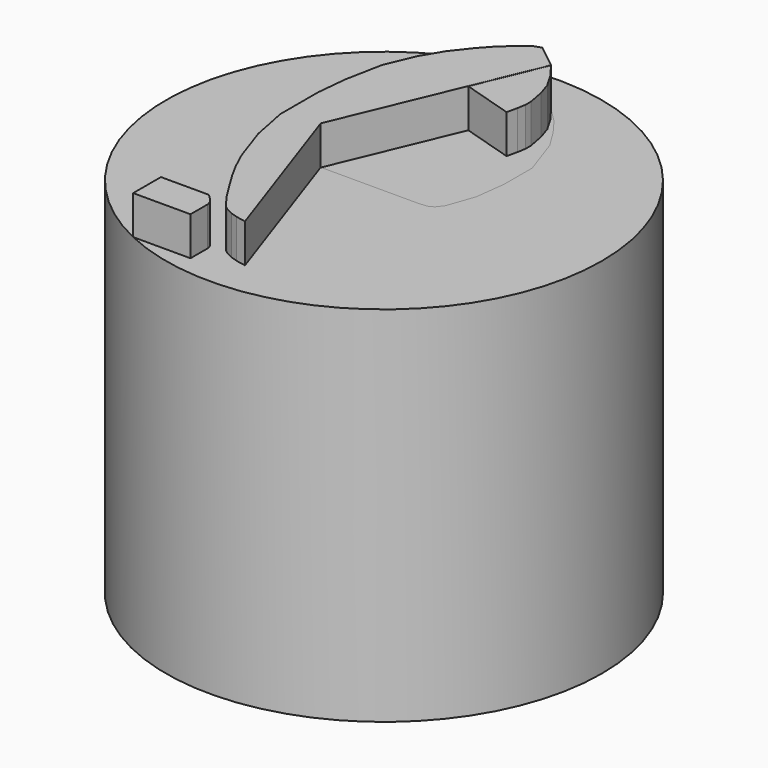
from build123d import *

# Parameters (mm, degrees)
F0_R     = 11.43
F1_DEPTH = 19.05
F4_DEPTH = 2.032
F5_DEPTH = 2.032
F7_DEPTH = 2.04216
F9_DEPTH = 2.032


# Not quite as in the source:
# - the program builds the solid bodies; features that only make, move or delete a surface that nothing else refers to are left out


with BuildPart() as f1:
    # F0 (on Top) → F1 (new body)
    with BuildSketch(Plane.XY):
        Circle(F0_R)
    extrude(amount=F1_DEPTH)

    # F2 (on face) → F4 (join)
    with BuildSketch(Plane.XY.offset(19.05)):
        Polygon((-1.880699303, -9.8758544773), (-1.880699303, -9.2042507604), (-1.9244262949, -9.0331919491), (-1.9849389791, -8.9233731851), (-2.1037228871, -8.7844179943), (-2.2359541617, -8.6320163682), (-2.3368084803, -8.5490914062), (-2.4040446151, -8.5124997422), (-4.8866966505, -8.5124997422), (-4.8866966505, -10.3327196733), (-1.880699303, -10.3327196733), align=None)
    extrude(amount=F4_DEPTH)

    # F3 (on face) → F5 (join)
    with BuildSketch(Plane.XY.offset(19.05)):
        Polygon((-1.7278705491, -8.1480639055), (-1.2155624572, -8.848301135), (-0.99472492, -9.0333931148), (-0.6215886096, -9.2146312818), (-0.2580773879, -9.3326671917), (0.2562761689, -9.4326803476), (-2.7548340149, -0.7004765794), (2.3825464305, -0.7004765794), (2.8303356376, -0.6551945116), (3.0876482706, -0.5188287272), (3.3525165636, -0.1815205032), (3.8505939301, 1.2300182134), (4.0490847188, 2.823865274), (4.0490847188, 3.8342506159), (4.0490847188, 4.6603621612), (3.7003470565, 5.6716995562), (3.3525165636, 6.6804061644), (2.7548240032, 7.6480992138), (2.1429003682, 8.4734838456), (1.3896959743, 9.2225758454), (0.4744292394, 9.9412809361), (0.1303268877, 10.2114842576), (-0.2051776682, 10.0957928225), (-0.6890241057, 9.7257923335), (-1.3436399167, 9.1707920656), (-1.9814397674, 8.4734838456), (-2.7524866164, 7.4915601872), (-3.3928717021, 6.4100213349), (-4.0235333078, 4.9190376551), (-4.2040259577, 3.9907894097), (-4.4032568112, 2.966173226), (-4.5597953722, 1.3723261654), (-4.5597953722, 0.5327102263), (-4.5597953722, -0.4492135195), (-4.5597953722, -1.1038292432), (-4.4032568112, -1.8722912064), (-4.1837464389, -2.9998348066), (-3.9051796775, -3.8076769561), (-3.6632562988, -4.519215785), (-3.5209483467, -4.9319081008), (-3.0940251891, -5.8569088578), (-2.6955632493, -6.5826787613), (-2.1829206962, -7.4222944677), align=None)
    extrude(amount=F5_DEPTH)

    # F6 (on face) → F7 (cut)
    with BuildSketch(Plane.XY.offset(21.082)):
        Polygon((1.3896959743, 9.2225758454), (-2.7548340149, -0.7004765794), (2.3825464305, -0.7004765794), (2.8303356376, -0.6551945116), (3.0876482706, -0.5188287272), (3.3525165636, -0.1815205032), (3.8505939301, 1.2300182134), (4.0490847188, 2.823865274), (4.0490847188, 4.6603621612), (3.3525165636, 6.6804061644), (2.7548240032, 7.6480992138), (2.1429003682, 8.4734838456), align=None)
    extrude(amount=-F7_DEPTH, mode=Mode.SUBTRACT)

    # F8 (on face) → F9 (join)
    with BuildSketch(Plane.XY.offset(19.03984)):
        Polygon((1.94505778, 8.4734838456), (1.3896959743, 9.2225758454), (-0.0989583414, 5.6583611201), (2.5561635848, 4.8432974145), (2.6805696543, 5.3959228098), (2.7548240032, 5.8293724433), (2.7548240032, 6.2017086893), (2.5935345329, 7.0562646724), (2.3686850909, 7.748354692), align=None)
    extrude(amount=F9_DEPTH)


solid = f1.part
